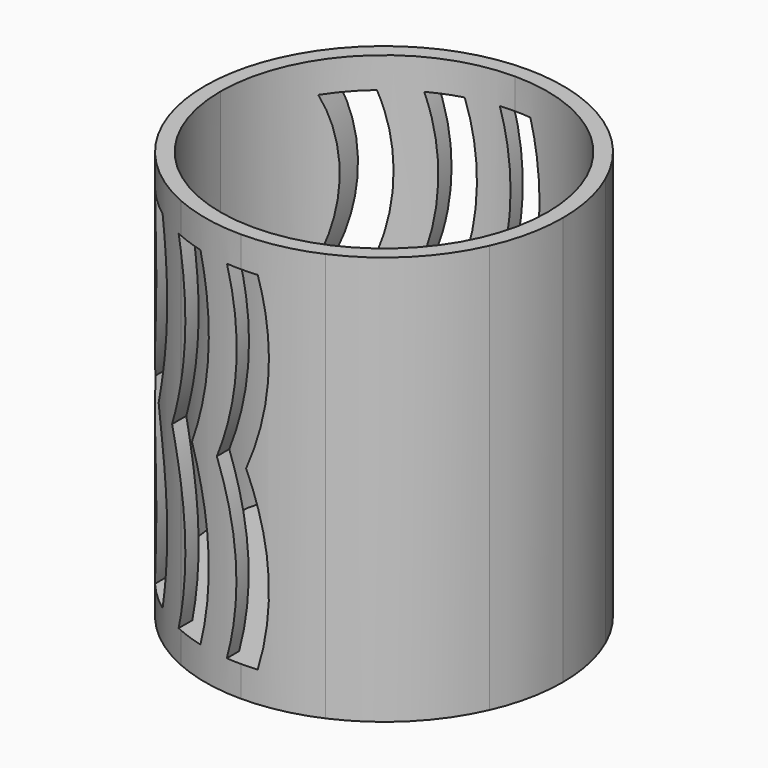
from build123d import *
from build123d import SkipClean  # not in build123d's __all__

# Parameters (mm, degrees)
F1_DEPTH = 7.62
F2_DEPTH = 101.6
F4_DEPTH = 88.901
F5_DEPTH = 101.6010001


with BuildPart() as f1:
    # F0 (on Top) → F1 (new body)
    with BuildSketch(Plane.XY):
        with BuildLine():
            ThreePointArc((0, -40.64), (28.7368195874, -28.7368195874), (40.64, 0))
            ThreePointArc((40.64, 0), (28.7368195874, 28.7368195874), (0, 40.64))
            Line((0, 40.64), (0, 0))
            Line((0, 0), (-40.64, 0))
            ThreePointArc((-40.64, 0), (-28.7368195874, -28.7368195874), (0, -40.64))
        make_face()
        with BuildLine():
            Line((0, 0), (0, 40.64))
            ThreePointArc((0, 40.64), (-28.7368195874, 28.7368195874), (-40.64, 0))
            Line((-40.64, 0), (0, 0))
        make_face()
    extrude(amount=F1_DEPTH)

    # F0 (on Top) → F2 (join)
    with BuildSketch(Plane.XY):
        with BuildLine():
            ThreePointArc((-18.005357536, 40.64), (-9.2020242338, 43.4870699174), (0, 44.45))
            Line((0, 44.45), (-44.45, 44.45))
            Line((-44.45, 44.45), (-44.45, 0))
            ThreePointArc((-44.45, 0), (-43.4870699174, 9.2020242338), (-40.64, 18.005357536))
            Line((-40.64, 18.005357536), (-40.64, 40.64))
            Line((-40.64, 40.64), (-18.005357536, 40.64))
        make_face()
        with BuildLine():
            Line((0, 40.64), (0, 44.45))
            ThreePointArc((0, 44.45), (-9.2020242338, 43.4870699174), (-18.005357536, 40.64))
            Line((-18.005357536, 40.64), (0, 40.64))
        make_face()
        with BuildLine():
            Line((0, 40.64), (18.005357536, 40.64))
            ThreePointArc((18.005357536, 40.64), (9.2020242338, 43.4870699174), (0, 44.45))
            Line((0, 44.45), (0, 40.64))
        make_face()
        with BuildLine():
            ThreePointArc((40.64, 18.005357536), (43.4870699174, 9.2020242338), (44.45, 0))
            Line((44.45, 0), (44.45, 44.45))
            Line((44.45, 44.45), (0, 44.45))
            ThreePointArc((0, 44.45), (9.2020242338, 43.4870699174), (18.005357536, 40.64))
            Line((18.005357536, 40.64), (40.64, 40.64))
            Line((40.64, 40.64), (40.64, 18.005357536))
        make_face()
        with BuildLine():
            ThreePointArc((40.64, -18.005357536), (43.4870699174, -9.2020242338), (44.45, 0))
            ThreePointArc((44.45, 0), (43.4870699174, 9.2020242338), (40.64, 18.005357536))
            Line((40.64, 18.005357536), (40.64, 0))
            Line((40.64, 0), (40.64, -18.005357536))
        make_face()
        with BuildLine():
            Line((44.45, -44.45), (44.45, 0))
            ThreePointArc((44.45, 0), (43.4870699174, -9.2020242338), (40.64, -18.005357536))
            Line((40.64, -18.005357536), (40.64, -40.64))
            Line((40.64, -40.64), (18.005357536, -40.64))
            ThreePointArc((18.005357536, -40.64), (9.2020243294, -43.4870698972), (1.953e-07, -44.45))
            Line((1.953e-07, -44.45), (44.45, -44.45))
        make_face()
        with BuildLine():
            ThreePointArc((1.953e-07, -44.45), (9.2020243294, -43.4870698972), (18.005357536, -40.64))
            Line((18.005357536, -40.64), (0, -40.64))
            Line((0, -40.64), (-18.005357536, -40.64))
            ThreePointArc((-18.005357536, -40.64), (-9.2020241383, -43.4870699376), (1.953e-07, -44.45))
        make_face()
        with BuildLine():
            Line((-44.45, 0), (-40.64, 0))
            Line((-40.64, 0), (-40.64, 18.005357536))
            ThreePointArc((-40.64, 18.005357536), (-43.4870699174, 9.2020242338), (-44.45, 0))
        make_face()
        with BuildLine():
            Line((-40.64, -18.005357536), (-40.64, 0))
            Line((-40.64, 0), (-44.45, 0))
            ThreePointArc((-44.45, 0), (-43.4870699174, -9.2020242338), (-40.64, -18.005357536))
        make_face()
        with BuildLine():
            Line((-44.45, -44.45), (1.953e-07, -44.45))
            ThreePointArc((1.953e-07, -44.45), (-9.2020241383, -43.4870699376), (-18.005357536, -40.64))
            Line((-18.005357536, -40.64), (-40.64, -40.64))
            Line((-40.64, -40.64), (-40.64, -18.005357536))
            ThreePointArc((-40.64, -18.005357536), (-43.4870699174, -9.2020242338), (-44.45, 0))
            Line((-44.45, 0), (-44.45, -44.45))
        make_face()
        with BuildLine():
            ThreePointArc((-40.64, 18.005357536), (-31.4308964237, 31.4308964237), (-18.005357536, 40.64))
            Line((-18.005357536, 40.64), (-40.64, 40.64))
            Line((-40.64, 40.64), (-40.64, 18.005357536))
        make_face()
        with BuildLine():
            ThreePointArc((18.005357536, 40.64), (31.4308964237, 31.4308964237), (40.64, 18.005357536))
            Line((40.64, 18.005357536), (40.64, 40.64))
            Line((40.64, 40.64), (18.005357536, 40.64))
        make_face()
        with BuildLine():
            Line((-40.64, -40.64), (-18.005357536, -40.64))
            ThreePointArc((-18.005357536, -40.64), (-31.4308964237, -31.4308964237), (-40.64, -18.005357536))
            Line((-40.64, -18.005357536), (-40.64, -40.64))
        make_face()
        with BuildLine():
            Line((40.64, -40.64), (40.64, -18.005357536))
            ThreePointArc((40.64, -18.005357536), (31.4308964237, -31.4308964237), (18.005357536, -40.64))
            Line((18.005357536, -40.64), (40.64, -40.64))
        make_face()
        with BuildLine():
            Line((40.64, 0), (40.64, 18.005357536))
            ThreePointArc((40.64, 18.005357536), (31.4308964237, 31.4308964237), (18.005357536, 40.64))
            Line((18.005357536, 40.64), (0, 40.64))
            ThreePointArc((0, 40.64), (28.7368195874, 28.7368195874), (40.64, 0))
        make_face()
        with BuildLine():
            ThreePointArc((-40.64, 0), (-28.7368195874, 28.7368195874), (0, 40.64))
            Line((0, 40.64), (-18.005357536, 40.64))
            ThreePointArc((-18.005357536, 40.64), (-31.4308964237, 31.4308964237), (-40.64, 18.005357536))
            Line((-40.64, 18.005357536), (-40.64, 0))
        make_face()
        with BuildLine():
            Line((-18.005357536, -40.64), (0, -40.64))
            ThreePointArc((0, -40.64), (-28.7368195874, -28.7368195874), (-40.64, 0))
            Line((-40.64, 0), (-40.64, -18.005357536))
            ThreePointArc((-40.64, -18.005357536), (-31.4308964237, -31.4308964237), (-18.005357536, -40.64))
        make_face()
        with BuildLine():
            ThreePointArc((18.005357536, -40.64), (31.4308964237, -31.4308964237), (40.64, -18.005357536))
            Line((40.64, -18.005357536), (40.64, 0))
            ThreePointArc((40.64, 0), (28.7368195874, -28.7368195874), (0, -40.64))
            Line((0, -40.64), (18.005357536, -40.64))
        make_face()
    extrude(amount=F2_DEPTH)

    # F3 (on face) → F4 (cut, through all)
    with BuildSketch(Plane.XZ.offset(44.45)):
        with BuildLine():
            Line((-26.4487113259, 93.98), (-34.0687113259, 93.98))
            ThreePointArc((-34.0687113259, 93.98), (-31.6581525371, 72.1475589103), (-36.83, 50.8))
            ThreePointArc((-36.83, 50.8), (-31.6581525371, 29.4524410897), (-34.0687113259, 7.62))
            Line((-34.0687113259, 7.62), (-26.4487113259, 7.62))
            ThreePointArc((-26.4487113259, 7.62), (-24.0381525371, 29.4524410897), (-29.21, 50.8))
            ThreePointArc((-29.21, 50.8), (-24.0381525371, 72.1475589103), (-26.4487113259, 93.98))
        make_face()
        with BuildLine():
            Line((-11.2087113259, 93.98), (-18.8287113259, 93.98))
            ThreePointArc((-18.8287113259, 93.98), (-16.4181525371, 72.1475589103), (-21.59, 50.8))
            ThreePointArc((-21.59, 50.8), (-16.4181525371, 29.4524410897), (-18.8287113259, 7.62))
            Line((-18.8287113259, 7.62), (-11.2087113259, 7.62))
            ThreePointArc((-11.2087113259, 7.62), (-8.7981525371, 29.4524410897), (-13.97, 50.8))
            ThreePointArc((-13.97, 50.8), (-8.7981525371, 72.1475589103), (-11.2087113259, 93.98))
        make_face()
        with BuildLine():
            Line((4.0312886741, 93.98), (-3.5887113259, 93.98))
            ThreePointArc((-3.5887113259, 93.98), (-1.1781525371, 72.1475589103), (-6.35, 50.8))
            ThreePointArc((-6.35, 50.8), (-1.2532449523, 29.4453529783), (-3.6306024792, 7.62))
            Line((-3.6306024792, 7.62), (4.0312886741, 7.62))
            ThreePointArc((4.0312886741, 7.62), (6.4418474629, 29.4524410897), (1.27, 50.8))
            ThreePointArc((1.27, 50.8), (6.4418474629, 72.1475589103), (4.0312886741, 93.98))
        make_face()
    extrude(amount=-F4_DEPTH, mode=Mode.SUBTRACT)

    # F0 (on Top) → F5 (cut, through all)
    with BuildSketch(Plane.XY):
        with BuildLine():
            Line((-44.45, -44.45), (1.953e-07, -44.45))
            ThreePointArc((1.953e-07, -44.45), (-9.2020241383, -43.4870699376), (-18.005357536, -40.64))
            Line((-18.005357536, -40.64), (-40.64, -40.64))
            Line((-40.64, -40.64), (-40.64, -18.005357536))
            ThreePointArc((-40.64, -18.005357536), (-43.4870699174, -9.2020242338), (-44.45, 0))
            Line((-44.45, 0), (-44.45, -44.45))
        make_face()
        with BuildLine():
            Line((-40.64, -40.64), (-18.005357536, -40.64))
            ThreePointArc((-18.005357536, -40.64), (-31.4308964237, -31.4308964237), (-40.64, -18.005357536))
            Line((-40.64, -18.005357536), (-40.64, -40.64))
        make_face()
        with BuildLine():
            ThreePointArc((-40.64, 18.005357536), (-31.4308964237, 31.4308964237), (-18.005357536, 40.64))
            Line((-18.005357536, 40.64), (-40.64, 40.64))
            Line((-40.64, 40.64), (-40.64, 18.005357536))
        make_face()
        with BuildLine():
            ThreePointArc((-18.005357536, 40.64), (-9.2020242338, 43.4870699174), (0, 44.45))
            Line((0, 44.45), (-44.45, 44.45))
            Line((-44.45, 44.45), (-44.45, 0))
            ThreePointArc((-44.45, 0), (-43.4870699174, 9.2020242338), (-40.64, 18.005357536))
            Line((-40.64, 18.005357536), (-40.64, 40.64))
            Line((-40.64, 40.64), (-18.005357536, 40.64))
        make_face()
        with BuildLine():
            ThreePointArc((18.005357536, 40.64), (31.4308964237, 31.4308964237), (40.64, 18.005357536))
            Line((40.64, 18.005357536), (40.64, 40.64))
            Line((40.64, 40.64), (18.005357536, 40.64))
        make_face()
        with BuildLine():
            ThreePointArc((40.64, 18.005357536), (43.4870699174, 9.2020242338), (44.45, 0))
            Line((44.45, 0), (44.45, 44.45))
            Line((44.45, 44.45), (0, 44.45))
            ThreePointArc((0, 44.45), (9.2020242338, 43.4870699174), (18.005357536, 40.64))
            Line((18.005357536, 40.64), (40.64, 40.64))
            Line((40.64, 40.64), (40.64, 18.005357536))
        make_face()
        with BuildLine():
            Line((40.64, -40.64), (40.64, -18.005357536))
            ThreePointArc((40.64, -18.005357536), (31.4308964237, -31.4308964237), (18.005357536, -40.64))
            Line((18.005357536, -40.64), (40.64, -40.64))
        make_face()
        with BuildLine():
            Line((44.45, -44.45), (44.45, 0))
            ThreePointArc((44.45, 0), (43.4870699174, -9.2020242338), (40.64, -18.005357536))
            Line((40.64, -18.005357536), (40.64, -40.64))
            Line((40.64, -40.64), (18.005357536, -40.64))
            ThreePointArc((18.005357536, -40.64), (9.2020243294, -43.4870698972), (1.953e-07, -44.45))
            Line((1.953e-07, -44.45), (44.45, -44.45))
        make_face()
    with SkipClean():  # cleaning this boolean's faces spoils the solid; the shape is the same uncleaned
        extrude(amount=F5_DEPTH, mode=Mode.SUBTRACT)


solid = f1.part
